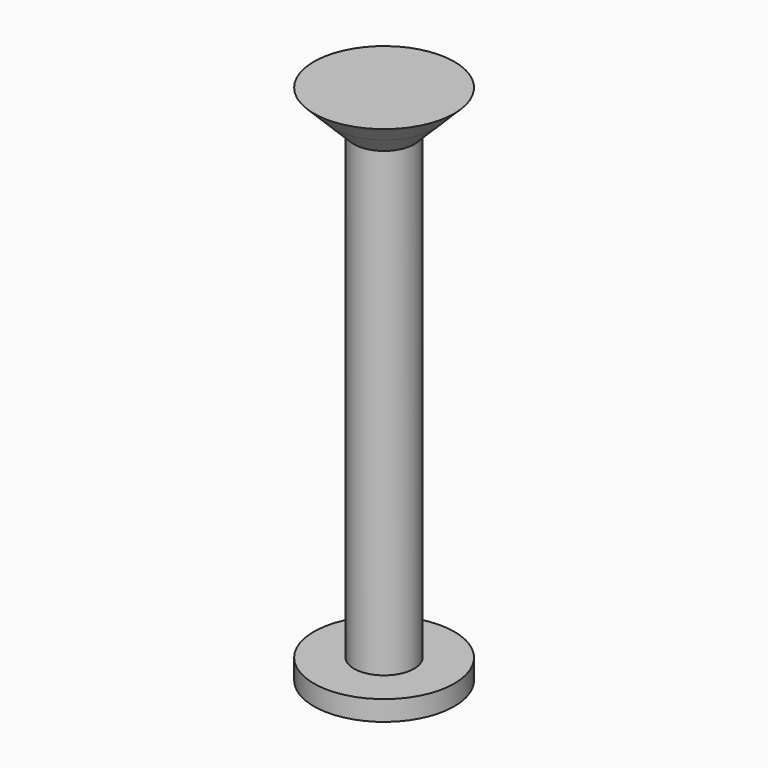
from build123d import *

# Parameters (mm, degrees)
F0_W    = 7.5
F0_H    = 120
F4_SIZE = 4.99999


# Not quite as in the source:
# - a fillet or chamfer is up to 0.001 mm smaller than in the source, because OpenCascade refuses the exact size


with BuildPart() as f1:
    # F0 (on Front) → F1 (revolve)
    with BuildSketch(Plane.XZ):
        Polygon((0, 65), (0, 60), (7.5, 60), (17.5, 60), (17.5, 65), align=None)
    revolve(axis=Axis((0, 0, 0), (0, 0, -1)))

    # F0 (on Front) → F2 (revolve)
    with BuildSketch(Plane.XZ):
        with Locations((3.75, 0)):
            Rectangle(F0_W, F0_H)
    revolve(axis=Axis((0, 0, 0), (0, 0, -1)))

    # F0 (on Front) → F3 (revolve)
    with BuildSketch(Plane.XZ):
        Polygon((7.5, -60), (0, -60), (0, -65), (17.5, -65), (17.5, -60), align=None)
    revolve(axis=Axis((0, 0, 0), (0, 0, -1)))

    # F4 (size 5 in the source; OpenCascade refuses exactly that, so slightly less here)
    f4_edges = [f1.edges().sort_by_distance(p)[0] for p in [
        (-17.5, 0, 60),
        (-7.5, 0, 60),
    ]]
    chamfer(f4_edges, length=F4_SIZE)


solid = f1.part
